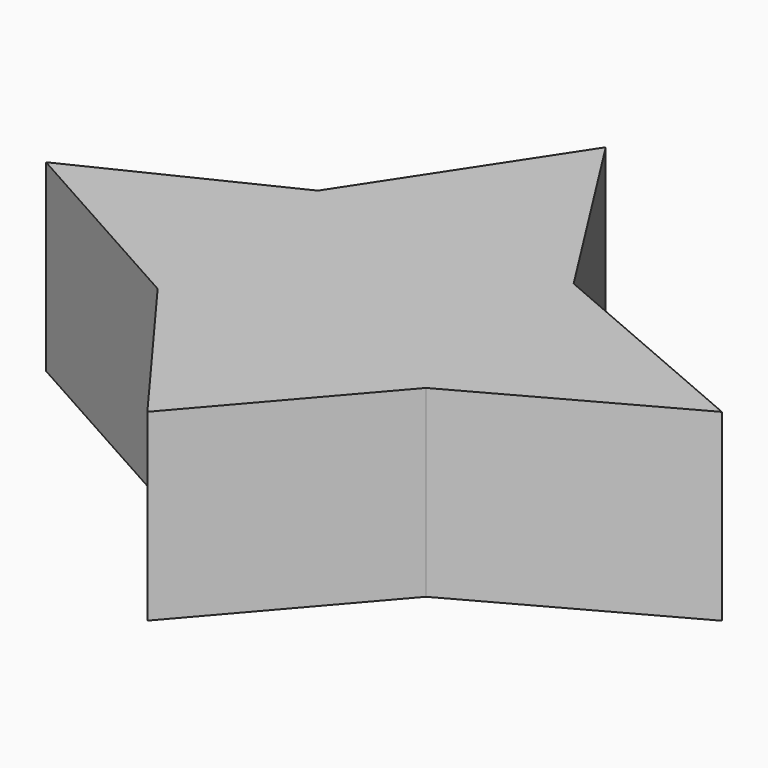
from build123d import *

# Parameters (mm, degrees)
F2_DEPTH = 25.4


# Not quite as in the source:
# - a feature of the source that left no trace in its solid (it failed there, or was rolled back) is left out


with BuildPart() as f2:
    # F1 (on face) → F2 (new body)
    with BuildSketch(Plane.XY):
        Polygon((0, 40.4482856393), (-17.9194230586, 13.1359212101), (-44.9530929327, 0), (-17.0833300799, -15.5699327588), (0, -38.7018322945), (19.9834518135, -15.5699327588), (48.4106056392, 0), (17.1964745969, 13.4146194905), align=None)
    extrude(amount=F2_DEPTH)


solid = f2.part
